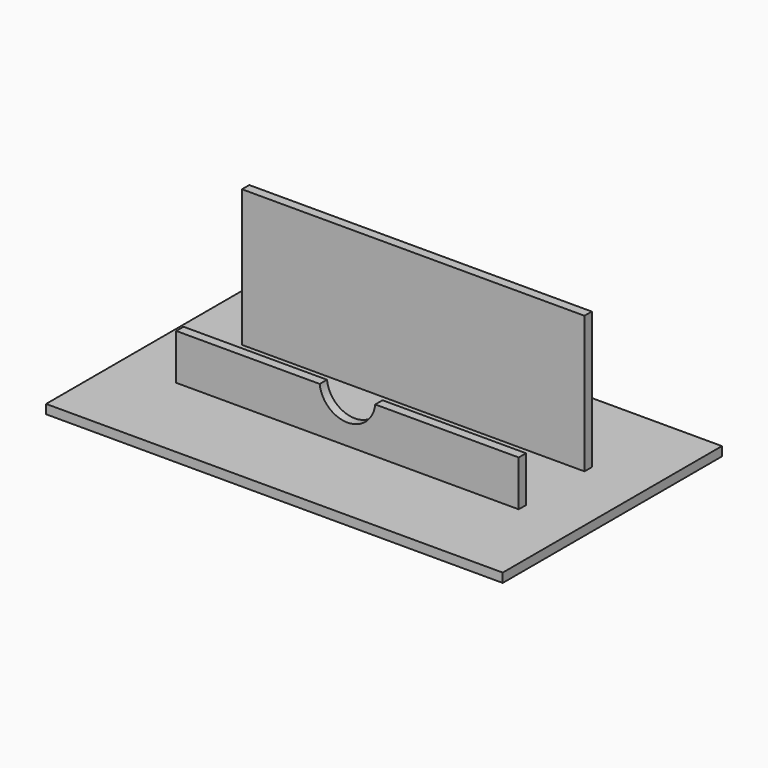
from build123d import *

# Parameters (mm, degrees)
F0_W        = 95.25
F0_H        = 25.4
F1_DEPTH    = 12.7
F2_W        = 127
F2_H        = 76.2
F3_DEPTH    = 2.54
F4_T        = 2.54
F4_T3_DEPTH = 100.33
F4_T5_DEPTH = 30.48
F5_DEPTH    = 25.4
F6_DEPTH    = 25.4
F7_DEPTH    = 25.4
F10_DEPTH   = 5.08


# Not quite as in the source:
# - a shell that OpenCascade refuses in one call is made with other operations: the cavity is built on its own and cut out


with BuildPart() as f1:
    # F0 (on Top) → F1 (new body)
    with BuildSketch(Plane.XY):
        Rectangle(F0_W, F0_H)
    extrude(amount=F1_DEPTH)

    # F2 (on Top) → F3 (join)
    with BuildSketch(Plane.XY):
        Rectangle(F2_W, F2_H)
    extrude(amount=-F3_DEPTH)

    # F4: shell of thickness 2.54, made by hand


with BuildPart() as f4_core1:
    # F4_t2: copy of F1
    add(f1.part)

    # the walls: a layer under each face that stays
    f4_faces = [f4_core1.faces().sort_by_distance(p)[0] for p in [
        (63.5, 0, -1.27),
        (0, -38.1, -1.27),
        (0, 38.1, -1.27),
        (-42.3333333333, -25.4, 0),
        (0, 0, -2.54),
        (-63.5, 0, -1.27),
        (0, -12.7, 6.35),
        (47.625, 0, 6.35),
        (0, 12.7, 6.35),
        (-47.625, 0, 6.35),
    ]]
    thicken(f4_faces, amount=-F4_T, mode=Mode.SUBTRACT)

    # F4_s4 → F4_t3 (cut)
    with BuildSketch(Plane.YZ.offset(-50.165)):
        Polygon((-12.7254, 0.0254), (-12.7, -2.54), (-10.16, -2.54), (-10.16, 0), align=None)
        Polygon((12.7254, 0.0254), (12.7, -2.54), (10.16, -2.54), (10.16, 0), align=None)
    extrude(amount=F4_T3_DEPTH, mode=Mode.SUBTRACT)

    # F4_s6 → F4_t5 (cut)
    with BuildSketch(Plane.XZ.offset(-15.24)):
        Polygon((47.6504, 0.0254), (47.625, -2.54), (45.085, -2.54), (45.085, 0), align=None)
        Polygon((-47.6504, 0.0254), (-47.625, -2.54), (-45.085, -2.54), (-45.085, 0), align=None)
    extrude(amount=F4_T5_DEPTH, mode=Mode.SUBTRACT)


with BuildPart() as f1_1:
    add(f1.part)

    # what is left inside the walls is the cavity
    f4_cavity = [f4_core1.part.solids().sort_by_distance(p)[0] for p in [
        (0, -3.386667, 0.0254),
    ]]
    add(f4_cavity, mode=Mode.SUBTRACT)

    # F5 (cut): a face of the model
    f5_faces = [f1_1.faces().sort_by_distance(p)[0] for p in [
        (-45.085, 0, 6.35),
    ]]
    extrude(f5_faces, amount=-F5_DEPTH, mode=Mode.SUBTRACT)

    # F6 (cut): a face of the model
    f6_faces = [f1_1.faces().sort_by_distance(p)[0] for p in [
        (45.085, 0, 6.35),
    ]]
    extrude(f6_faces, amount=-F6_DEPTH, mode=Mode.SUBTRACT)

    # F7 (add): a face of the model
    f7_faces = [f1_1.faces().sort_by_distance(p)[0] for p in [
        (0, 11.43, 12.7),
    ]]
    extrude(f7_faces, amount=F7_DEPTH)

    # F9 (on face) → F10 (cut)
    with BuildSketch(Plane.XZ.offset(12.7)):
        with BuildLine():
            ThreePointArc((7.7229928646, 12.7), (7.7554155926, 13.1086234281), (7.7662332139, 13.5183883831))
            ThreePointArc((7.7662332139, 13.5183883831), (-0.409764955, 21.2738039757), (-7.7229928646, 12.7))
            Line((-7.7229928646, 12.7), (7.7229928646, 12.7))
        make_face()
        with BuildLine():
            Line((7.7229928646, 12.7), (-7.7229928646, 12.7))
            ThreePointArc((-7.7229928646, 12.7), (0, 5.7521551692), (7.7229928646, 12.7))
        make_face()
    extrude(amount=-F10_DEPTH, mode=Mode.SUBTRACT)


solid = f1_1.part
